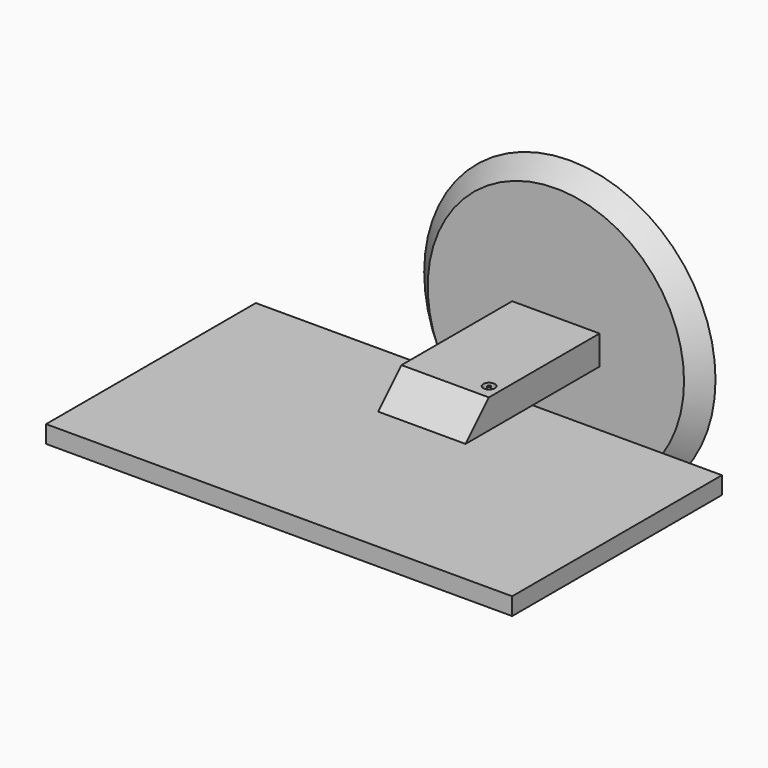
from build123d import *

# Parameters (mm, degrees)
F0_R      = 50
F1_DEPTH  = 6
F2_SIZE   = 5.99999
F4_DEPTH  = 57.5
F5_W      = 15
F5_H      = 28.75
F6_DEPTH  = 6
F7_W      = 154
F7_H      = 78
F8_DEPTH  = 1
F9_SIZE   = 9.99999
F10_R     = 2.2025754481
F11_DEPTH = 0.3
F12_DEPTH = 0.35
F13_R     = 2
F13_R_2   = 0.5
F14_DEPTH = 2


# Not quite as in the source:
# - a fillet or chamfer is up to 0.001 mm smaller than in the source, because OpenCascade refuses the exact size


with BuildPart() as f1:
    # F0 (on Front) → F1 (new body)
    with BuildSketch(Plane.XZ):
        with Locations((-39.6165661514, 33.0943278968)):
            Circle(F0_R)
    extrude(amount=F1_DEPTH)

    # F2 (size 6 in the source; OpenCascade refuses exactly that, so slightly less here)
    f2_edges = [f1.edges().sort_by_distance(p)[0] for p in [
        (-89.616566, -6, 33.094328),
    ]]
    chamfer(f2_edges, length=F2_SIZE)

    # F3 (on face) → F4 (join)
    with BuildSketch(Plane.XZ.offset(6)):
        Polygon((-54.6165661514, 28.0943278968), (-39.6165661514, 28.0943278968), (-24.6165661514, 28.0943278968), (-24.6165661514, 38.0943278968), (-39.6165661514, 38.0943278968), (-54.6165661514, 38.0943278968), align=None)
    extrude(amount=F4_DEPTH)

    # F5 (on face) → F6 (join)
    with BuildSketch(Plane(origin=(0, 0, 28.0943278968), x_dir=(1, 0, 0), z_dir=(0, 0, -1))):
        Polygon((-119.6165661514, 34.75), (-54.6165661514, 34.75), (-54.6165661514, 63.5), (-39.6165661514, 63.5), (-24.6165661514, 63.5), (-24.6165661514, 34.75), (40.3834338486, 34.75), (40.3834338486, 124.75), (-39.6165661514, 124.75), (-119.6165661514, 124.75), align=None)
        with Locations((-32.1165661514, 49.125)):
            Rectangle(F5_W, F5_H)
        with Locations((-47.1165661514, 49.125)):
            Rectangle(F5_W, F5_H)
    extrude(amount=F6_DEPTH)

    # F7 (on face) → F8 (cut)
    with BuildSketch(Plane(origin=(0, 0, 22.0943278968), x_dir=(1, 0, 0), z_dir=(0, 0, -1))):
        with Locations((-39.6165661514, 82.5612554252)):
            Rectangle(F7_W, F7_H)
    extrude(amount=-F8_DEPTH, mode=Mode.SUBTRACT)

    # F9 (size 10 in the source; OpenCascade refuses exactly that, so slightly less here)
    f9_edges = [f1.edges().sort_by_distance(p)[0] for p in [
        (-39.616566, -63.5, 38.094328),
    ]]
    chamfer(f9_edges, length=F9_SIZE)

    # F10 (on face) → F11 (join)
    with BuildSketch(Plane(origin=(0, 0, 22.0943278968), x_dir=(1, 0, 0), z_dir=(0, 0, -1))):
        with Locations((32.0070236921, 39.2166003585)):
            Circle(F10_R)
        with BuildLine():
            ThreePointArc((33.2229098133, 40.4324864797), (32.0070236921, 37.4970777156), (30.7911375709, 40.4324864797))
            ThreePointArc((30.7911375709, 40.4324864797), (31.1349833923, 40.4324864797), (31.1349833923, 40.0886406584))
            ThreePointArc((31.1349833923, 40.0886406584), (32.0070236921, 37.9833491395), (32.879063992, 40.0886406584))
            ThreePointArc((32.879063992, 40.0886406584), (32.879063992, 40.4324864797), (33.2229098133, 40.4324864797))
        make_face(mode=Mode.SUBTRACT)
        with BuildLine():
            ThreePointArc((32.2499889227, 39.2166003585), (32.0070236921, 38.9736351279), (31.7640584616, 39.2166003585))
            Line((31.7640584616, 39.2166003585), (31.7640584616, 40.6014584005))
            ThreePointArc((31.7640584616, 40.6014584005), (32.0070236921, 40.844423631), (32.2499889227, 40.6014584005))
            Line((32.2499889227, 40.6014584005), (32.2499889227, 39.2166003585))
        make_face(mode=Mode.SUBTRACT)
    extrude(amount=F11_DEPTH)

    # F12 (add): faces of the model
    f12_faces = [f1.faces().sort_by_distance(p)[0] for p in [
        (32.0070236921, -39.9090293795, 22.0943278968),
        (32.0070236921, -37.5427579145, 22.0943278968),
    ]]
    extrude(f12_faces, amount=F12_DEPTH)

    # F13 (on face) → F14 (cut)
    with BuildSketch(Plane.XY.offset(38.0943278968)):
        with Locations((-28.6587122828, -48.3524724841)):
            Circle(F13_R)
        with Locations((-28.6587122828, -48.3524724841)):
            Circle(F13_R_2, mode=Mode.SUBTRACT)
    extrude(amount=-F14_DEPTH, mode=Mode.SUBTRACT)


solid = f1.part
